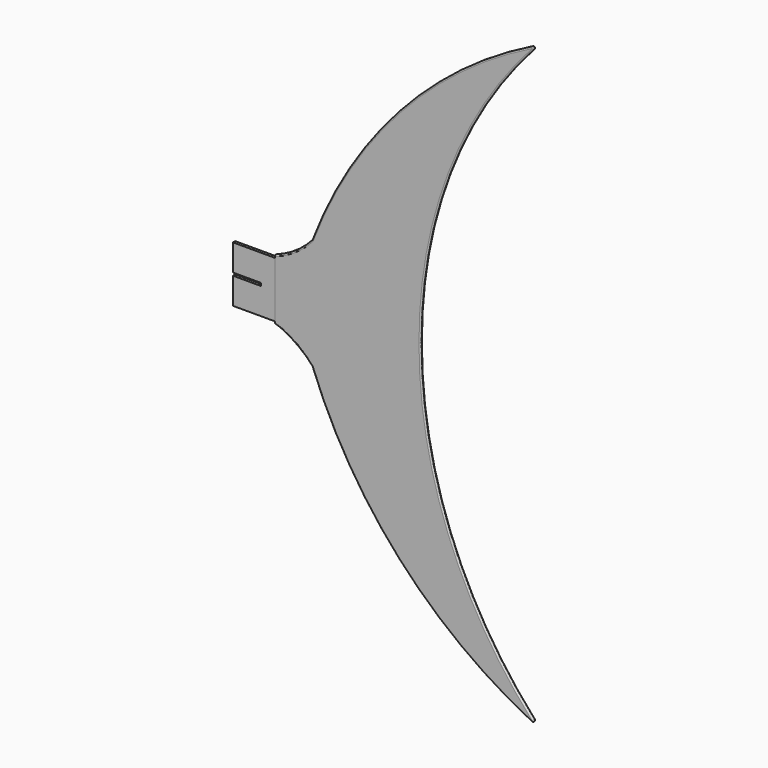
from build123d import *

# Parameters (mm, degrees)
F1_DEPTH = 0.5
F2_R     = 0.4999
F0_W     = 15
F0_H     = 10
F4_DEPTH = 0.5
F6_W     = 10
F6_H     = 1
F7_DEPTH = 1.0010001


# Not quite as in the source:
# - a fillet or chamfer is up to 0.001 mm smaller than in the source, because OpenCascade refuses the exact size


with BuildPart() as f1:
    # F0 (on Front) → F1 (new body, symmetric)
    with BuildSketch(Plane.XZ):
        with BuildLine():
            ThreePointArc((13.2612720792, 19.8919038619), (7.1998646271, 14.5536810673), (0, 10.8931848908))
            Line((0, 10.8931848908), (0, 10))
            Line((0, 10), (0, 0))
            Line((0, 0), (52.0978415222, 0))
            ThreePointArc((52.0978415222, 0), (62.8950817615, 57.7854744772), (94.2497236639, 107.511))
            ThreePointArc((94.2497236639, 107.511), (45.2820813919, 71.5336359019), (13.2612720792, 19.8919038619))
        make_face()
    extrude(amount=F1_DEPTH, both=True)

    # F2 (radius 0.5 in the source; OpenCascade refuses exactly that, so slightly less here)
    f2_edges = [f1.edges().sort_by_distance(p)[0] for p in [
        (7.199865, -0.5, 14.553681),
        (7.199865, 0.5, 14.553681),
        (45.282081, -0.5, 71.533636),
        (45.282081, 0.5, 71.533636),
        (13.261272, 0, 19.891904),
        (94.249724, 0, 107.511),
        (62.895082, 0.5, 57.785474),
        (62.895082, -0.5, 57.785474),
    ]]
    fillet(f2_edges, radius=F2_R)

    # F3: F1 across plane


with BuildPart() as f1_1:
    add(f1.part)
    add(f1.part.mirror(Plane.XY))


with BuildPart() as f4:
    # F0 (on Front) → F4 (new body, symmetric)
    with BuildSketch(Plane.XZ):
        with Locations((-7.5, 5)):
            Rectangle(F0_W, F0_H)
    extrude(amount=F4_DEPTH, both=True)

    # F5: F4 across plane


with BuildPart() as f4_1:
    add(f4.part)
    add(f4.part.mirror(Plane.XY))

    # F6 (on face) → F7 (cut, through all)
    with BuildSketch(Plane.XZ.offset(0.5)):
        with Locations((-10, 0)):
            Rectangle(F6_W, F6_H)
    extrude(amount=-F7_DEPTH, mode=Mode.SUBTRACT)


solid = Compound([f1_1.part, f4_1.part])
